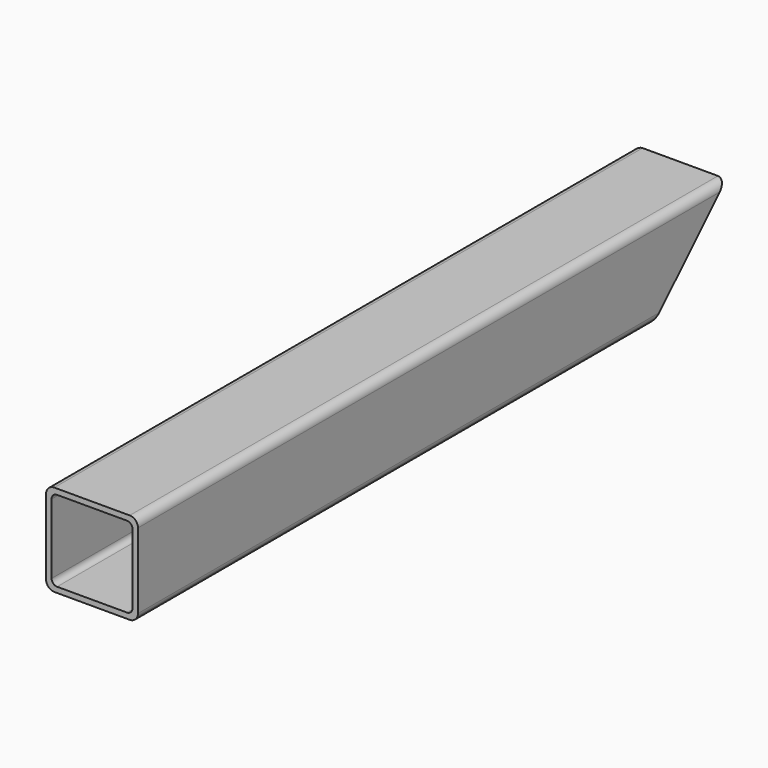
from build123d import *

# Parameters (mm, degrees)
F1_DEPTH = 400
F3_DEPTH = 50.001


# Not quite as in the source:
# - a feature names something its author has since deleted; it is built from what else it names


with BuildPart() as f1:
    # F0 (on Front) → F1 (new body)
    with BuildSketch(Plane.XZ):
        with BuildLine():
            Line((45.5, 0), (4.5, 0))
            ThreePointArc((4.5, 0), (1.3180194847, -1.3180194847), (0, -4.5))
            Line((0, -4.5), (0, -45.5))
            ThreePointArc((0, -45.5), (1.3180194847, -48.6819805153), (4.5, -50))
            Line((4.5, -50), (45.5, -50))
            ThreePointArc((45.5, -50), (48.6819805153, -48.6819805153), (50, -45.5))
            Line((50, -45.5), (50, -4.5))
            ThreePointArc((50, -4.5), (48.6819805153, -1.3180194847), (45.5, 0))
        make_face()
        with BuildLine():
            ThreePointArc((3, -6), (3.8786796564, -3.8786796564), (6, -3))
            Line((6, -3), (44, -3))
            ThreePointArc((44, -3), (46.1213203436, -3.8786796564), (47, -6))
            Line((47, -6), (47, -44))
            ThreePointArc((47, -44), (46.1213203436, -46.1213203436), (44, -47))
            Line((44, -47), (6, -47))
            ThreePointArc((6, -47), (3.8786796564, -46.1213203436), (3, -44))
            Line((3, -44), (3, -6))
        make_face(mode=Mode.SUBTRACT)
    extrude(amount=F1_DEPTH)

    # F2 (on Right) → F3 (cut, through all)
    with BuildSketch(Plane.YZ):
        Polygon((29.2893218813, 0), (0, 0), (-45.5, -45.5), (-70.7106781187, -70.7106781187), (29.2893218813, -70.7106781187), align=None)
    extrude(amount=F3_DEPTH, mode=Mode.SUBTRACT)


solid = f1.part
